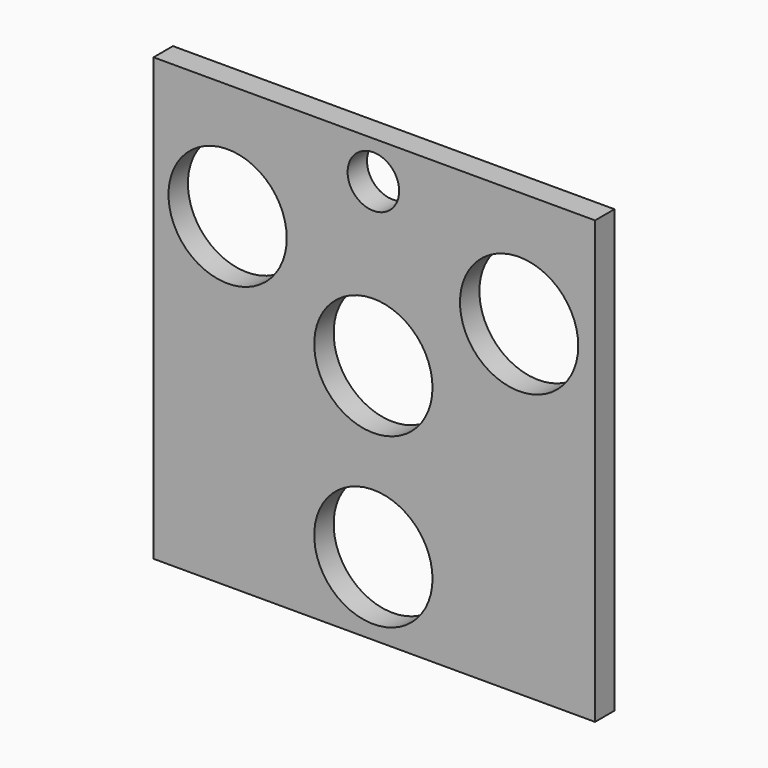
from build123d import *

# Parameters (mm, degrees)
F0_W      = 80
F0_H      = 120
F0_R      = 9.75
F0_R_2    = 4.25
F1_DEPTH  = 4
F3_W      = 80
F3_H      = 20
F4_DEPTH  = 10
F5_W      = 6
F5_H      = 6
F5_R      = 0.95
F6_DEPTH  = 10
F7_R      = 2.99999
F11_W     = 97.9346781969
F11_H     = 127.8536170721
F11_W_2   = 72.8027671576
F11_H_2   = 72.8027634323
F12_DEPTH = 10


# Not quite as in the source:
# - a fillet or chamfer is up to 0.001 mm smaller than in the source, because OpenCascade refuses the exact size


with BuildPart() as f1:
    # F0 (on Front) → F1 (new body)
    with BuildSketch(Plane.XZ):
        Rectangle(F0_W, F0_H)
        with Locations((0, -24.624)):
            Circle(F0_R, mode=Mode.SUBTRACT)
        with Locations((-24.032204955, 17.001)):
            Circle(F0_R, mode=Mode.SUBTRACT)
        with Locations((0, 3.126)):
            Circle(F0_R, mode=Mode.SUBTRACT)
        with Locations((0, 29.876)):
            Circle(F0_R_2, mode=Mode.SUBTRACT)
        with Locations((24.032204955, 17.001)):
            Circle(F0_R, mode=Mode.SUBTRACT)
    extrude(amount=F1_DEPTH)

    # F3 (on face) → F4 (cut)
    with BuildSketch(Plane.XZ.offset(4)):
        with Locations((0, -50)):
            Rectangle(F3_W, F3_H)
    extrude(amount=-F4_DEPTH, mode=Mode.SUBTRACT)

    # F8: F6 across plane


with BuildPart() as f6:
    # F5 (on face) → F6 (new body)
    with BuildSketch(Plane.XZ.offset(4)):
        with Locations((43, 3)):
            Rectangle(F5_W, F5_H)
        with Locations((42.5, 3.126)):
            Circle(F5_R, mode=Mode.SUBTRACT)
    extrude(amount=-F6_DEPTH)

    # F7 (radius 3 in the source; OpenCascade refuses exactly that, so slightly less here)
    f7_edges = [f6.edges().sort_by_distance(p)[0] for p in [
        (46, 1, 0),
        (46, 1, 6),
    ]]
    fillet(f7_edges, radius=F7_R)


with BuildPart() as f1_1:
    add(f1.part)
    add(f6.part.mirror(Plane.YZ))


with BuildPart() as f12_tool:
    # F11 (on face) → F12 (new body)
    with BuildSketch(Plane.XZ.offset(4)):
        with Locations((1.1506490409, -1.4746189117)):
            Rectangle(F11_W, F11_H)
        with Locations((0.1533515751, -0.2778600901)):
            Rectangle(F11_W_2, F11_H_2, mode=Mode.SUBTRACT)
    extrude(amount=-F12_DEPTH)


with BuildPart() as f1_2:
    add(f1_1.part)

    # F12: cut by f12_tool
    add(f12_tool.part, mode=Mode.SUBTRACT)


with BuildPart() as f6_1:
    add(f6.part)

    # F12: cut by f12_tool
    add(f12_tool.part, mode=Mode.SUBTRACT)


solid = f1_2.part
